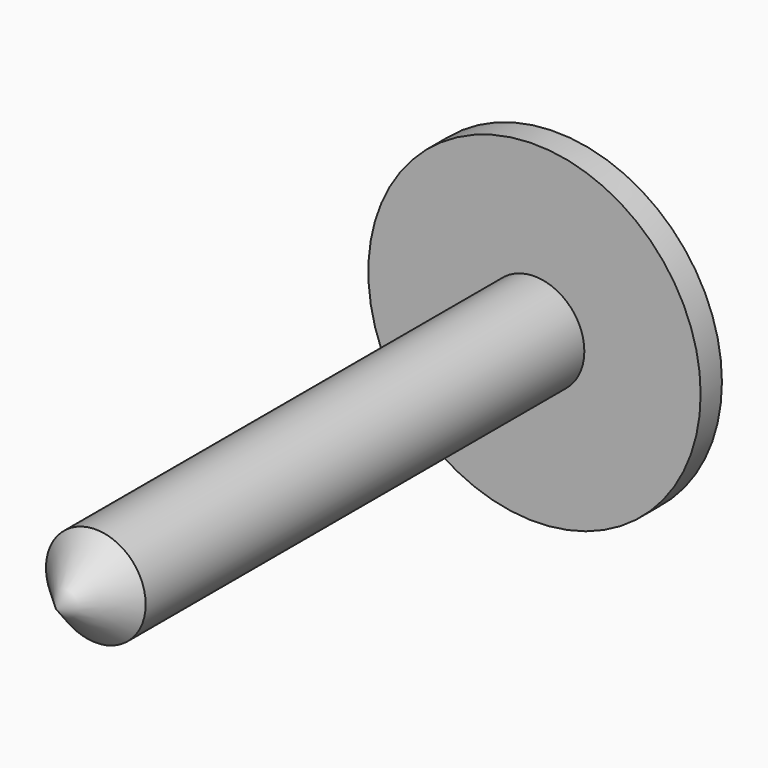
from build123d import *

# Parameters (mm, degrees)
F0_R            = 12.5
F1_DEPTH        = 2
F2_R            = 3.75
F3_DEPTH        = 45
F4_SIZE         = 3.75
F7_DEPTH        = 0.5
F7_COPIES_COUNT = 20


# Not quite as in the source:
# - a pattern or mirror of a feature is missing from the dataset's text; its kind, count and spacing are read off the source's solid


with BuildPart() as f1:
    # F0 (on Front) → F1 (new body)
    with BuildSketch(Plane.XZ):
        Circle(F0_R)
    extrude(amount=F1_DEPTH)

    # F2 (on face) → F3 (join)
    with BuildSketch(Plane.XZ.offset(2)):
        Circle(F2_R)
    extrude(amount=F3_DEPTH)

    # F4
    f4_edges = [f1.edges().sort_by_distance(p)[0] for p in [
        (-3.75, -47, 0),
    ]]
    chamfer(f4_edges, length=F4_SIZE)

    # F6 (on Front) → F7 (cut)
    with BuildSketch(Plane.XZ):
        with BuildLine():
            Line((-0.5, 3.85), (0.5, 3.85))
            Line((0.5, 3.85), (0.5, 11.4891252931))
            ThreePointArc((0.5, 11.4891252931), (0, 11.5), (-0.5, 11.4891252931))
            Line((-0.5, 11.4891252931), (-0.5, 3.85))
        make_face()
    f7 = extrude(amount=F7_DEPTH, mode=Mode.SUBTRACT)

    # F7_copies: F7 ×20 about axis
    f7_copies_axis = Axis((0, 0, 0), (0, 1, 0))
    for i in range(1, F7_COPIES_COUNT):
        add(f7.rotate(f7_copies_axis, i * 360 / F7_COPIES_COUNT), mode=Mode.SUBTRACT)


solid = f1.part
